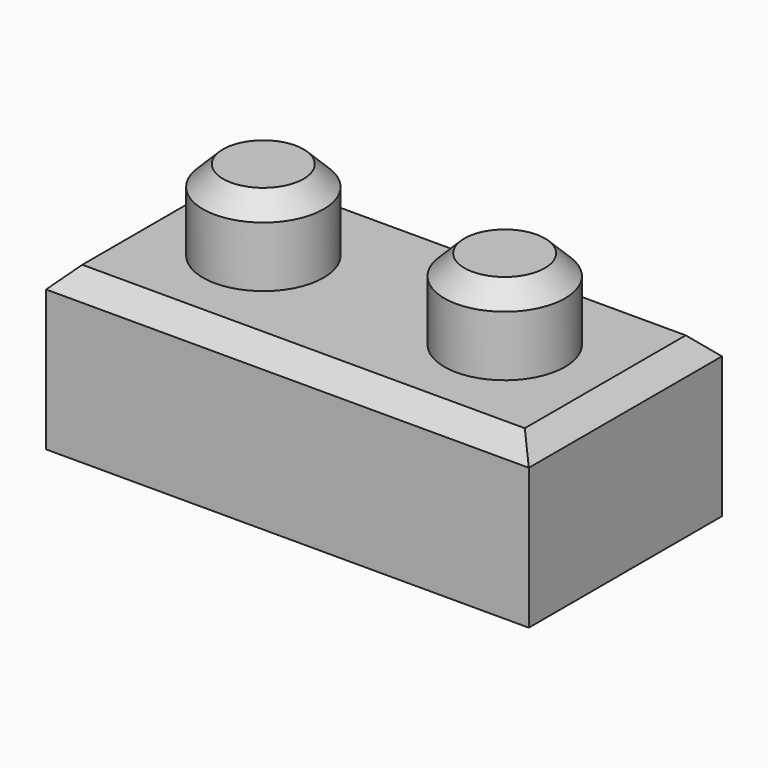
from build123d import *

# Parameters (mm, degrees)
F0_W     = 76.2
F0_H     = 38.1
F1_DEPTH = 25.4
F2_SIZE  = 3.175
F3_R     = 9.525
F4_DEPTH = 12.7
F5_SIZE2 = 3.175
F5_SIZE  = 3.175
F6_T     = 7.9375


# Not quite as in the source:
# - a shell that OpenCascade refuses in one call is made with other operations: the cavity is built on its own and cut out


with BuildPart() as f1:
    # F0 (on Top) → F1 (new body)
    with BuildSketch(Plane.XY):
        with Locations((38.1, -19.05)):
            Rectangle(F0_W, F0_H)
    extrude(amount=F1_DEPTH)

    # F2
    f2_edges = [f1.edges().sort_by_distance(p)[0] for p in [
        (38.1, -38.1, 25.4),
        (76.2, -19.05, 25.4),
        (38.1, 0, 25.4),
        (0, -19.05, 25.4),
    ]]
    chamfer(f2_edges, length=F2_SIZE)

    # F3 (on face) → F4 (join)
    with BuildSketch(Plane.XY.offset(25.4)):
        with Locations((19.05, -19.05)):
            Circle(F3_R)
        with Locations((57.15, -19.05)):
            Circle(F3_R)
    extrude(amount=F4_DEPTH)

    # F5
    f5_edges = [f1.edges().sort_by_distance(p)[0] for p in [
        (9.525, -19.05, 38.1),
        (47.625, -19.05, 38.1),
    ]]
    chamfer(f5_edges, length=F5_SIZE, length2=F5_SIZE2)

    # F6: shell of thickness 7.9375, made by hand


with BuildPart() as f6_core1:
    # F6_t2: copy of F1
    add(f1.part)

    # the walls: a layer under each face that stays
    f6_faces = [f6_core1.faces().sort_by_distance(p)[0] for p in [
        (9.525, -19.05, 30.1625),
        (11.1125, -19.05, 36.5125),
        (38.1, -19.05, 25.4),
        (19.05, -19.05, 38.1),
        (38.1, -36.5125, 23.8125),
        (1.5875, -19.05, 23.8125),
        (74.6125, -19.05, 23.8125),
        (38.1, -1.5875, 23.8125),
        (47.625, -19.05, 30.1625),
        (38.1, -38.1, 11.1125),
        (0, -19.05, 11.1125),
        (76.2, -19.05, 11.1125),
        (38.1, 0, 11.1125),
        (49.2125, -19.05, 36.5125),
        (57.15, -19.05, 38.1),
    ]]
    thicken(f6_faces, amount=-F6_T, mode=Mode.SUBTRACT)

    # F6_s3 → F6_t4 (revolve, cut)
    with BuildSketch(Plane.XZ.offset(19.05)):
        Polygon((28.654375, 25.479375), (20.6375, 25.4), (20.6375, 17.4625), (28.575, 17.4625), align=None)
    revolve(axis=Axis((19.05, -19.05, 25.4), (0, 0, 1)), mode=Mode.SUBTRACT)

    # F6_s5 → F6_t6 (revolve, cut)
    with BuildSketch(Plane.XZ.offset(19.05)):
        Polygon((66.754375, 25.479375), (66.675, 17.4625), (58.7375, 17.4625), (58.7375, 25.4), align=None)
    revolve(axis=Axis((57.15, -19.05, 25.4), (0, 0, 1)), mode=Mode.SUBTRACT)


with BuildPart() as f1_1:
    add(f1.part)

    # what is left inside the walls is the cavity
    f6_cavity = [f6_core1.part.solids().sort_by_distance(p)[0] for p in [
        (38.1, -22.754167, 0.079375),
    ]]
    add(f6_cavity, mode=Mode.SUBTRACT)


solid = f1_1.part
